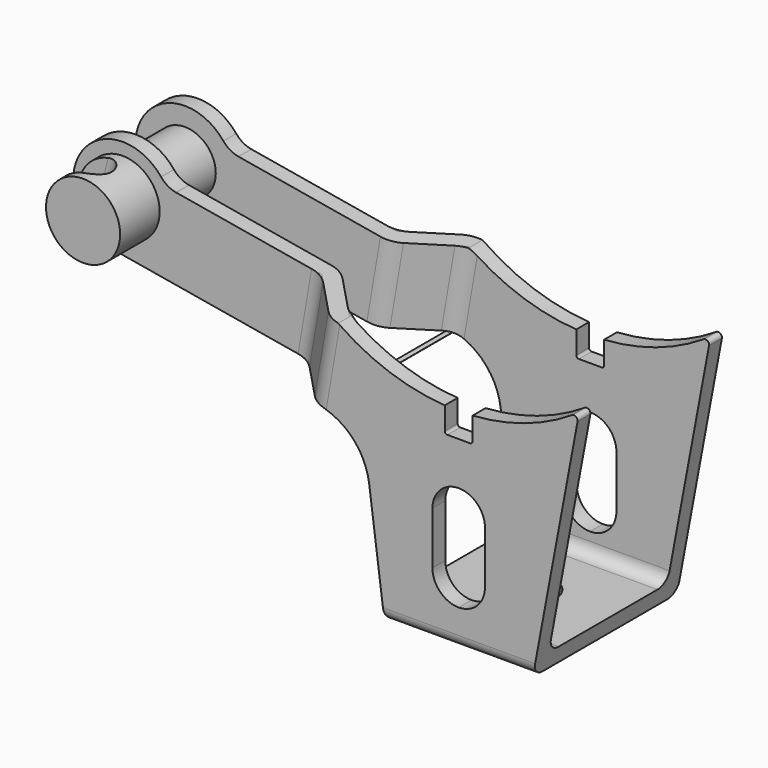
from build123d import *

# Parameters (mm, degrees)
F1_DEPTH       = 7.3
F1_DEPTH_BACK  = 7.3
F3_DEPTH       = 6
F3_DEPTH_BACK  = 6
F5_DEPTH       = 10
F5_DEPTH_BACK  = 10
F8_DEPTH       = 25
F9_R           = 2.5
F10_DEPTH      = 2.5
F10_DEPTH_BACK = 2.5
F11_T1_DEPTH   = 6.5
F11_T6_DEPTH   = 12.7132034356
F11_S7_R       = 5
F11_T8_DEPTH   = 8
F11_S10_R      = 17
F11_T11_DEPTH  = 8
F11_T15_DEPTH  = 8.5710678119
F11_T20_DEPTH  = 12.7132034356
F11_S21_R      = 5
F11_T22_DEPTH  = 8
F11_S24_R      = 17
F11_T25_DEPTH  = 8
F11_T29_DEPTH  = 8.5710678119
F11_T31_DEPTH  = 10.6421356237
F12_R          = 1
F13_R          = 2
F14_DEPTH      = 5
F15_R          = 1.05
F16_DEPTH      = 3
F16_DEPTH_BACK = 10
F17_SIZE       = 1
F19_START      = 3.8
F18_R          = 3
F19_DEPTH      = 4
F21_START      = 4.5
F21_DEPTH      = 2.6
F22_R          = 1.29999


# Not quite as in the source:
# - a fillet or chamfer that OpenCascade refuses, or shapes differently, is made with other operations: its cross-section is extruded or revolved along the edge and cut away or added
# - a fillet or chamfer is up to 0.001 mm smaller than in the source, because OpenCascade refuses the exact size


with BuildPart() as f1:
    # F0 (on Front) → F1 (new body, two sides)
    with BuildSketch(Plane.XZ) as f1_sk:
        with BuildLine():
            Line((-7.2480415045, 9.479816391), (-6, 0))
            Line((-6, 0), (6, 0))
            Line((6, 0), (9.6197658273, 19.3731186918))
            ThreePointArc((9.6197658273, 19.3731186918), (9.492555749, 19.6769779623), (9.1631662961, 19.6809084286))
            ThreePointArc((9.1631662961, 19.6809084286), (-0.3536100614, 17.0036780472), (-9.750799418, 20.0744152471))
            Line((-9.750799418, 20.0744152471), (-25.666835692, 22.7954629152))
            ThreePointArc((-25.666835692, 22.7954629152), (-26.3420622378, 23.0419468668), (-26.8865335991, 23.511240126))
            ThreePointArc((-26.8865335991, 23.511240126), (-33.4498266444, 23.0245236782), (-30.6740705867, 17.0572054525))
            Line((-30.6740705867, 17.0572054525), (-11.362677578, 13.7556786143))
            ThreePointArc((-11.362677578, 13.7556786143), (-8.6024605414, 12.2941429125), (-7.2480415045, 9.479816391))
        make_face()
    extrude(amount=F1_DEPTH)
    extrude(f1_sk.sketch, amount=-F1_DEPTH_BACK)

    # F2 (on Front) → F3 (cut, two sides)
    with BuildSketch(Plane.XZ) as f3_sk:
        Polygon((15, 1.3), (15, 78.0352148958), (0, 78.0352148958), (-11, 13.6936742961), (-11, 1.3), align=None)
    extrude(amount=F3_DEPTH, mode=Mode.SUBTRACT)
    extrude(f3_sk.sketch, amount=-F3_DEPTH_BACK, mode=Mode.SUBTRACT)

    # F4 (on Front) → F5 (cut, two sides)
    with BuildSketch(Plane.XZ) as f5_sk:
        with BuildLine():
            Line((0, 18), (-1.125, 18))
            Line((-1.125, 18), (-1.125, 15.2))
            ThreePointArc((-1.125, 15.2), (-1.0664213562, 15.0585786438), (-0.925, 15))
            Line((-0.925, 15), (0, 15))
            Line((0, 15), (0.925, 15))
            ThreePointArc((0.925, 15), (1.0664213562, 15.0585786438), (1.125, 15.2))
            Line((1.125, 15.2), (1.125, 18))
            Line((1.125, 18), (0, 18))
        make_face()
        with BuildLine():
            ThreePointArc((0, 11.5), (-1.50260191, 10.87760191), (-2.125, 9.375))
            Line((-2.125, 9.375), (-2.125, 5.125))
            ThreePointArc((-2.125, 5.125), (-1.50260191, 3.62239809), (0, 3))
            ThreePointArc((0, 3), (1.50260191, 3.62239809), (2.125, 5.125))
            Line((2.125, 5.125), (2.125, 9.375))
            ThreePointArc((2.125, 9.375), (1.50260191, 10.87760191), (0, 11.5))
        make_face()
    extrude(amount=F5_DEPTH, mode=Mode.SUBTRACT)
    extrude(f5_sk.sketch, amount=-F5_DEPTH_BACK, mode=Mode.SUBTRACT)

    # F7 (on offset) → F8 (cut)
    with BuildSketch(Plane(origin=(1.9622434031, 0, 11.4776148716), x_dir=(0.9856986369, 0, -0.1685176467), z_dir=(-0.1685176467, 0, -0.9856986369))):
        Polygon((-41.9907133171, -7.3), (-13.6887884036, -7.3), (-17.1887884036, -3.8), (-41.9907133171, -3.8), align=None)
        Polygon((-41.9907133171, 7.3), (-41.9907133171, 3.8), (-17.1887884036, 3.8), (-13.6887884036, 7.3), align=None)
        Polygon((-16.6503107725, -2.5), (-13.1503107725, -6), (-13.1503107725, 0), (-13.1503107725, 6), (-16.6503107725, 2.5), (-41.9907133171, 2.5), (-41.9907133171, 0), (-41.9907133171, -2.5), align=None)
    extrude(amount=-F8_DEPTH, mode=Mode.SUBTRACT)

    # F9 (on Front) → F10 (join, two sides)
    with BuildSketch(Plane.XZ) as f10_sk:
        with Locations((-30, 21)):
            Circle(F9_R)
    extrude(amount=F10_DEPTH)
    extrude(f10_sk.sketch, amount=-F10_DEPTH_BACK)

    # F11: fillet of radius 2 on 8 edges, made by hand

    # F11_s2 → F11_t1 (join)
    with BuildSketch(Plane(origin=(1.9622434031, 0, 11.4776148716), x_dir=(0, 1, 0), z_dir=(0.1685176467, 0, 0.9856986369))):
        with BuildLine():
            ThreePointArc((3.8, 18.0172155284), (3.952240935, 17.2518486636), (4.3857864376, 16.603001966))
            Line((4.3857864376, 16.603001966), (3.8, 17.1887884036))
            Line((3.8, 17.1887884036), (3.8, 18.0172155284))
        make_face()
        with BuildLine():
            ThreePointArc((-4.3857864376, 16.603001966), (-3.952240935, 17.2518486636), (-3.8, 18.0172155284))
            Line((-3.8, 18.0172155284), (-3.8, 17.1887884036))
            Line((-3.8, 17.1887884036), (-4.3857864376, 16.603001966))
        make_face()
    extrude(amount=F11_T1_DEPTH)


with BuildPart() as f11_tool4:
    # F11_s5 → F11_t6 (new body)
    with BuildSketch(Plane(origin=(3.0576081065, 0, 17.8846560114), x_dir=(0, 1, 0), z_dir=(-0.1685176467, 0, -0.9856986369))):
        with BuildLine():
            ThreePointArc((-6, -12.3218836478), (-5.847759065, -13.0872505125), (-5.4142135624, -13.7360972102))
            Line((-5.4142135624, -13.7360972102), (-6, -13.1503107725))
            Line((-6, -13.1503107725), (-6, -12.3218836478))
        make_face()
    extrude(amount=F11_T6_DEPTH)

    # F11_s7 → F11_t8 (cut, symmetric)
    with BuildSketch(Plane.XZ.offset(5.7)):
        with Locations((-12.2052658114, 8.8271854299)):
            Circle(F11_S7_R)
    extrude(amount=F11_T8_DEPTH, both=True, mode=Mode.SUBTRACT)

    split(bisect_by=Plane.YZ.offset(-11), keep=Keep.TOP)

    # F11_s10 → F11_t11 (cut, symmetric)
    with BuildSketch(Plane.XZ.offset(5.7)):
        with Locations((0, 34)):
            Circle(F11_S10_R)
    extrude(amount=F11_T11_DEPTH, both=True, mode=Mode.SUBTRACT)


with BuildPart() as f1_1:
    add(f1.part)

    # F11_t3: union F11_tool4
    add(f11_tool4.part)


with BuildPart() as f11_tool13:
    # F11_s14 → F11_t15 (new body)
    with BuildSketch(Plane(origin=(3.4066195803, 0, 19.9261047304), x_dir=(0, 1, 0), z_dir=(-0.1685176467, 0, -0.9856986369))):
        with BuildLine():
            ThreePointArc((-6, -12.3218836478), (-5.847759065, -13.0872505125), (-5.4142135624, -13.7360972102))
            Line((-5.4142135624, -13.7360972102), (-6, -13.1503107725))
            Line((-6, -13.1503107725), (-6, -12.3218836478))
        make_face()
    extrude(amount=F11_T15_DEPTH)

    split(bisect_by=Plane.YZ.offset(-11), keep=Keep.BOTTOM)


with BuildPart() as f1_2:
    add(f1_1.part)

    # F11_t12: union F11_tool13
    add(f11_tool13.part)


with BuildPart() as f11_tool18:
    # F11_s19 → F11_t20 (new body)
    with BuildSketch(Plane(origin=(3.0576081065, 0, 17.8846560114), x_dir=(0, 1, 0), z_dir=(-0.1685176467, 0, -0.9856986369))):
        with BuildLine():
            ThreePointArc((6, -12.3218836478), (5.847759065, -13.0872505125), (5.4142135624, -13.7360972102))
            Line((5.4142135624, -13.7360972102), (6, -13.1503107725))
            Line((6, -13.1503107725), (6, -12.3218836478))
        make_face()
    extrude(amount=F11_T20_DEPTH)

    # F11_s21 → F11_t22 (cut, symmetric)
    with BuildSketch(Plane.XZ.offset(-5.7)):
        with Locations((-12.2052658114, 8.8271854299)):
            Circle(F11_S21_R)
    extrude(amount=F11_T22_DEPTH, both=True, mode=Mode.SUBTRACT)

    split(bisect_by=Plane.YZ.offset(-11), keep=Keep.TOP)

    # F11_s24 → F11_t25 (cut, symmetric)
    with BuildSketch(Plane.XZ.offset(-5.7)):
        with Locations((0, 34)):
            Circle(F11_S24_R)
    extrude(amount=F11_T25_DEPTH, both=True, mode=Mode.SUBTRACT)


with BuildPart() as f1_3:
    add(f1_2.part)

    # F11_t17: union F11_tool18
    add(f11_tool18.part)


with BuildPart() as f11_tool27:
    # F11_s28 → F11_t29 (new body)
    with BuildSketch(Plane(origin=(3.4066195803, 0, 19.9261047304), x_dir=(0, 1, 0), z_dir=(-0.1685176467, 0, -0.9856986369))):
        with BuildLine():
            ThreePointArc((6, -12.3218836478), (5.847759065, -13.0872505125), (5.4142135624, -13.7360972102))
            Line((5.4142135624, -13.7360972102), (6, -13.1503107725))
            Line((6, -13.1503107725), (6, -12.3218836478))
        make_face()
    extrude(amount=F11_T29_DEPTH)

    split(bisect_by=Plane.YZ.offset(-11), keep=Keep.BOTTOM)


with BuildPart() as f1_4:
    add(f1_3.part)

    # F11_t26: union F11_tool27
    add(f11_tool27.part)

    # F11_s32 → F11_t31 (cut)
    with BuildSketch(Plane(origin=(1.6132319293, 0, 9.4361661525), x_dir=(0, 1, 0), z_dir=(0.1685176467, 0, 0.9856986369))):
        with BuildLine():
            ThreePointArc((6.7142135624, 14.2745748413), (7.147759065, 13.6257281436), (7.3, 12.8603612789))
            Line((7.3, 12.8603612789), (7.3, 13.6887884036))
            Line((7.3, 13.6887884036), (6.7142135624, 14.2745748413))
        make_face()
        with BuildLine():
            ThreePointArc((-2.5, 17.4787378973), (-2.652240935, 16.7133710326), (-3.0857864376, 16.0645243349))
            Line((-3.0857864376, 16.0645243349), (-2.5, 16.6503107725))
            Line((-2.5, 16.6503107725), (-2.5, 17.4787378973))
        make_face()
        with BuildLine():
            ThreePointArc((-6.7142135624, 14.2745748413), (-7.147759065, 13.6257281436), (-7.3, 12.8603612789))
            Line((-7.3, 12.8603612789), (-7.3, 13.6887884036))
            Line((-7.3, 13.6887884036), (-6.7142135624, 14.2745748413))
        make_face()
        with BuildLine():
            ThreePointArc((2.5, 17.4787378973), (2.652240935, 16.7133710326), (3.0857864376, 16.0645243349))
            Line((3.0857864376, 16.0645243349), (2.5, 16.6503107725))
            Line((2.5, 16.6503107725), (2.5, 17.4787378973))
        make_face()
    extrude(amount=F11_T31_DEPTH, mode=Mode.SUBTRACT)

    # F12
    f12_edges = [f1_4.edges().sort_by_distance(p)[0] for p in [
        (0.035875, 6, 1.3),
        (0, -7.3, 0),
        (0.035875, -6, 1.3),
        (0, 7.3, 0),
    ]]
    fillet(f12_edges, radius=F12_R)

    # F13 (on Top) → F14 (cut)
    with BuildSketch(Plane.XY):
        Circle(F13_R)
    extrude(amount=F14_DEPTH, mode=Mode.SUBTRACT)

    # F15 (on Front) → F16 (cut, two sides)
    with BuildSketch(Plane.XZ) as f16_sk:
        with Locations((-30, 21)):
            Circle(F15_R)
    extrude(amount=F16_DEPTH, mode=Mode.SUBTRACT)
    extrude(f16_sk.sketch, amount=-F16_DEPTH_BACK, mode=Mode.SUBTRACT)

    # F17
    f17_edges = [f1_4.edges().sort_by_distance(p)[0] for p in [
        (-31.05, 3.8, 21),
    ]]
    chamfer(f17_edges, length=F17_SIZE)

    # F18 (on Front) → F19 (join)
    with BuildSketch(Plane.XZ.offset(F19_START)):
        with Locations((-30, 21)):
            Circle(F18_R)
    extrude(amount=F19_DEPTH)

    # F20 (on Front) → F21 (cut)
    with BuildSketch(Plane.XZ.offset(F21_START)):
        Polygon((-40.5470757535, 15.9000791133), (-31.814414217, 13.7227820529), (-28.185585783, 28.2772179471), (-36.9182473195, 30.4545150075), align=None)
    extrude(amount=F21_DEPTH, mode=Mode.SUBTRACT)

    # F22 (radius 1.3 in the source; OpenCascade refuses exactly that, so slightly less here)
    f22_edges = [f1_4.edges().sort_by_distance(p)[0] for p in [
        (-30, -4.5, 21),
        (-30, -7.1, 21),
    ]]
    fillet(f22_edges, radius=F22_R)


solid = f1_4.part
